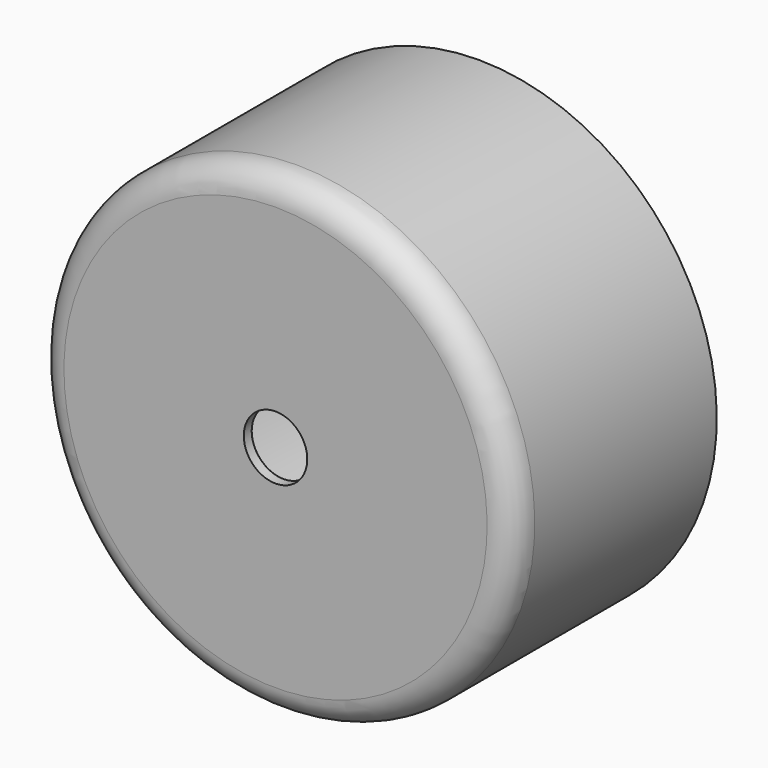
from build123d import *

# Parameters (mm, degrees)
F2_W        = 22
F2_H        = 42
F2_W_2      = 16
F2_H_2      = 36
F3_DEPTH    = 2
F2_R        = 6
F4_DEPTH    = 25
F5_T1_DEPTH = 14.5024142536
F6_R        = 0.5
F7_R        = 0.2


# Not quite as in the source:
# - a fillet or chamfer that OpenCascade refuses, or shapes differently, is made with other operations: its cross-section is extruded or revolved along the edge and cut away or added


with BuildPart() as f1:
    # F0 (on Right) → F1 (revolve)
    with BuildSketch(Plane.YZ):
        with BuildLine():
            Line((-23, 0), (-21, 0))
            Line((-21, 0), (-21, 32.1))
            Line((-21, 32.1), (-21, 34.1))
            Line((-21, 34.1), (-21, 40))
            ThreePointArc((-21, 40), (-20.1213203436, 42.1213203436), (-18, 43))
            Line((-18, 43), (15, 43))
            Line((15, 43), (17, 43))
            Line((17, 43), (23, 43))
            Line((23, 43), (25, 43))
            Line((25, 43), (25, 45))
            Line((25, 45), (-18, 45))
            ThreePointArc((-18, 45), (-21.5355339059, 43.5355339059), (-23, 40))
            Line((-23, 40), (-23, 0))
        make_face()
    revolve(axis=Axis((0, -22, 0), (0, -1, 0)))

    # F2 (on face) → F3 (join)
    with BuildSketch(Plane(origin=(0, -21, 0), x_dir=(-1, 0, 0), z_dir=(0, 1, 0))):
        Rectangle(F2_W, F2_H)
        Rectangle(F2_W_2, F2_H_2, mode=Mode.SUBTRACT)
    extrude(amount=F3_DEPTH)

    # F2 (on face) → F4 (cut)
    with BuildSketch(Plane(origin=(0, -21, 0), x_dir=(-1, 0, 0), z_dir=(0, 1, 0))):
        Circle(F2_R)
    extrude(amount=-F4_DEPTH, mode=Mode.SUBTRACT)

    # F5: fillet of radius 5 on 4 edges, made by hand

    # F5_s2 → F5_t1 (cut)
    with BuildSketch(Plane.XZ.offset(6.4975857464)):
        with BuildLine():
            ThreePointArc((5.9990343146, 21.0004), (9.5355339059, 19.5355339059), (11.0004, 15.9990343146))
            Line((11.0004, 15.9990343146), (11.5005365685, 15.9990343146))
            ThreePointArc((11.5005365685, 15.9990343146), (11.5001365685, 18.4995171573), (11.5001365685, 21))
            Line((11.5001365685, 21), (11, 21.5001365685))
            ThreePointArc((11, 21.5001365685), (8.4995171573, 21.5001365685), (5.9990343146, 21.5005365685))
            Line((5.9990343146, 21.5005365685), (5.9990343146, 21.0004))
        make_face()
        with BuildLine():
            ThreePointArc((-5.9990343146, 21.0004), (-9.5355339059, 19.5355339059), (-11.0004, 15.9990343146))
            Line((-11.0004, 15.9990343146), (-11.5005365685, 15.9990343146))
            ThreePointArc((-11.5005365685, 15.9990343146), (-11.5001365685, 18.4995171573), (-11.5001365685, 21))
            Line((-11.5001365685, 21), (-11, 21.5001365685))
            ThreePointArc((-11, 21.5001365685), (-8.4995171573, 21.5001365685), (-5.9990343146, 21.5005365685))
            Line((-5.9990343146, 21.5005365685), (-5.9990343146, 21.0004))
        make_face()
        with BuildLine():
            ThreePointArc((-5.9990343146, -21.0004), (-9.5355339059, -19.5355339059), (-11.0004, -15.9990343146))
            Line((-11.0004, -15.9990343146), (-11.5005365685, -15.9990343146))
            ThreePointArc((-11.5005365685, -15.9990343146), (-11.5001365685, -18.4995171573), (-11.5001365685, -21))
            Line((-11.5001365685, -21), (-11, -21.5001365685))
            ThreePointArc((-11, -21.5001365685), (-8.4995171573, -21.5001365685), (-5.9990343146, -21.5005365685))
            Line((-5.9990343146, -21.5005365685), (-5.9990343146, -21.0004))
        make_face()
        with BuildLine():
            ThreePointArc((11.0004, -15.9990343146), (9.5355339059, -19.5355339059), (5.9990343146, -21.0004))
            Line((5.9990343146, -21.0004), (5.9990343146, -21.5005365685))
            ThreePointArc((5.9990343146, -21.5005365685), (8.4995171573, -21.5001365685), (11, -21.5001365685))
            Line((11, -21.5001365685), (11.5001365685, -21))
            ThreePointArc((11.5001365685, -21), (11.5001365685, -18.4995171573), (11.5005365685, -15.9990343146))
            Line((11.5005365685, -15.9990343146), (11.0004, -15.9990343146))
        make_face()
    extrude(amount=F5_T1_DEPTH, mode=Mode.SUBTRACT)

    # F6
    f6_edges = [f1.edges().sort_by_distance(p)[0] for p in [
        (0, -21, -40),
        (0, -21, 21),
        (-9.535534, -21, 19.535534),
        (-11, -21, 0),
        (-9.535534, -21, -19.535534),
        (0, -21, -21),
        (9.535534, -21, -19.535534),
        (11, -21, 0),
        (9.535534, -21, 19.535534),
    ]]
    fillet(f6_edges, radius=F6_R)

    # F7
    f7_edges = [f1.edges().sort_by_distance(p)[0] for p in [
        (8, -21, 0),
        (0, -21, -18),
        (0, -21, 18),
        (-8, -21, 0),
        (6, -21, 0),
        (0, -21, -40),
    ]]
    fillet(f7_edges, radius=F7_R)


solid = f1.part
